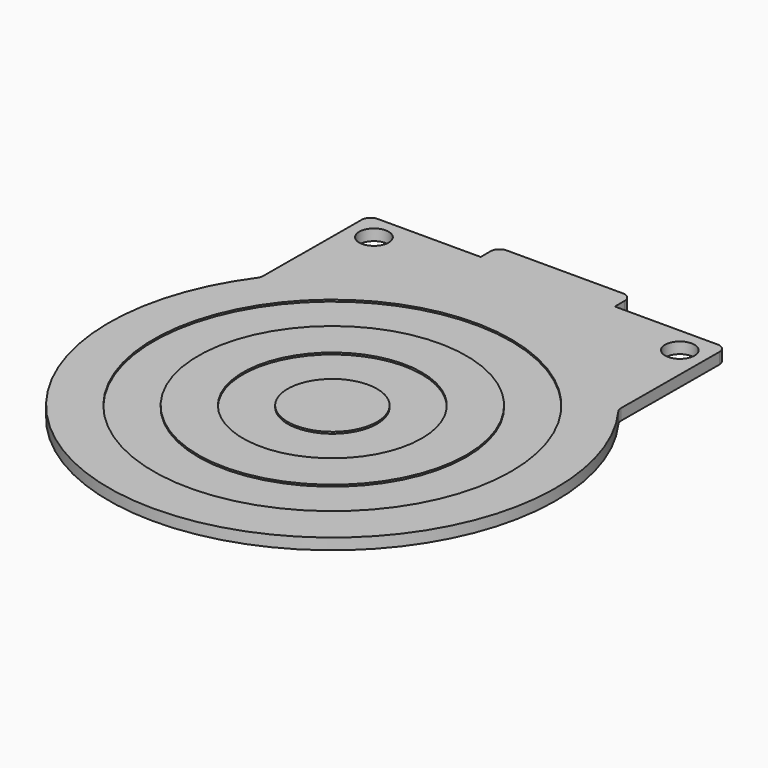
from build123d import *

# Parameters (mm, degrees)
F0_R     = 38.1
F0_R_2   = 25.4
F1_DEPTH = 3.175
F0_R_3   = 12.7
F0_R_4   = 50.8
F0_R_5   = 4.191
F2_DEPTH = 2.667
F3_R     = 2.54


# Not quite as in the source:
# - a feature names something its author has since deleted; it is built from what else it names


with BuildPart() as f1:
    # F0 (on Top) → F1 (new body)
    with BuildSketch(Plane.XY):
        Circle(F0_R)
        Circle(F0_R_2, mode=Mode.SUBTRACT)
    extrude(amount=F1_DEPTH)


with BuildPart() as f1b:
    # F0 (on Top) → F1, piece 2 (new body)
    with BuildSketch(Plane.XY):
        Circle(F0_R_3)
    extrude(amount=F1_DEPTH)


with BuildPart() as f1c:
    # F0 (on Top) → F1, piece 3 (new body)
    with BuildSketch(Plane.XY):
        with BuildLine():
            Line((-50.5914217212, 76.1994290653), (-50.8, 38.1))
            ThreePointArc((-50.8, 38.1), (0, -63.5), (50.8, 38.1))
            Line((50.8, 38.1), (51.0085782789, 76.1994290653))
            Line((51.0085782789, 76.1994290653), (19.2585782788, 76.1994290653))
            Line((19.2585782788, 76.1994290653), (19.2585782788, 82.256702956))
            Line((19.2585782788, 82.256702956), (-18.8414217212, 82.256702956))
            Line((-18.8414217212, 82.256702956), (-18.8414217212, 76.1994290653))
            Line((-18.8414217212, 76.1994290653), (-50.5914217211, 76.1994290653))
        make_face()
        Circle(F0_R_4, mode=Mode.SUBTRACT)
        with Locations((-43.265636348, 68.8335622319)):
            Circle(F0_R_5, mode=Mode.SUBTRACT)
        with Locations((43.6021421583, 68.8334290653)):
            Circle(F0_R_5, mode=Mode.SUBTRACT)
    extrude(amount=F1_DEPTH)

    # F3
    f3_edges = [f1c.edges().sort_by_distance(p)[0] for p in [
        (-18.841422, 82.256703, 1.5875),
        (19.258578, 82.256703, 1.5875),
        (-50.591422, 76.199429, 1.5875),
        (51.008578, 76.199429, 1.5875),
        (-50.8, 38.1, 1.5875),
        (50.8, 38.1, 1.5875),
    ]]
    fillet(f3_edges, radius=F3_R)


with BuildPart() as f2:
    # F0 (on Top) → F2 (new body)
    with BuildSketch(Plane.XY):
        Circle(F0_R_4)
        Circle(F0_R, mode=Mode.SUBTRACT)
    extrude(amount=F2_DEPTH)


with BuildPart() as f2b:
    # F0 (on Top) → F2, piece 2 (new body)
    with BuildSketch(Plane.XY):
        Circle(F0_R_2)
        Circle(F0_R_3, mode=Mode.SUBTRACT)
    extrude(amount=F2_DEPTH)


solid = Compound([f1.part, f1b.part, f1c.part, f2.part, f2b.part])
